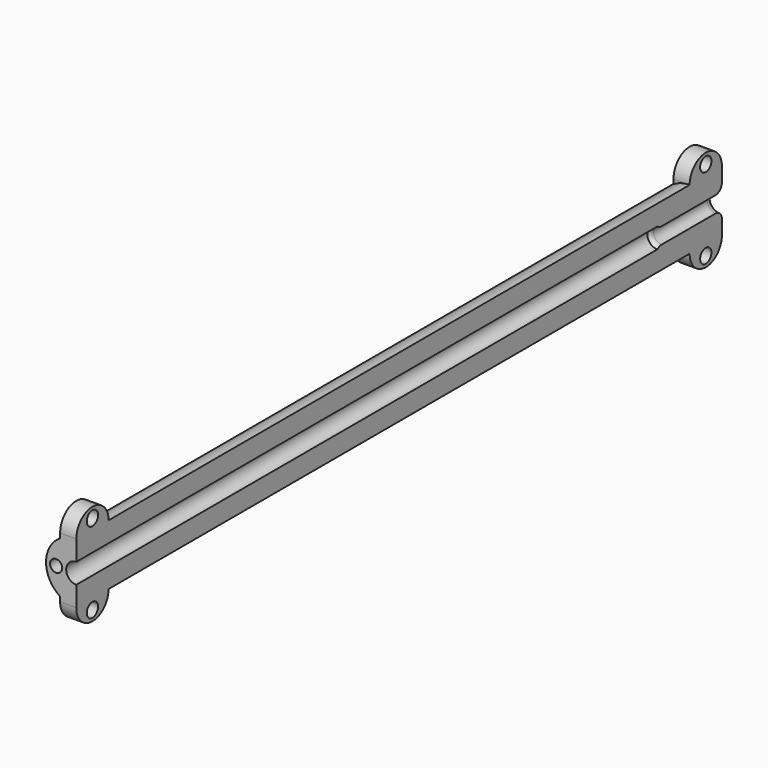
from build123d import *

# Parameters (mm, degrees)
F0_R         = 7.5
F0_R_2       = 2.5
F1_DEPTH     = 200
F2_R         = 1.5
F3_DEPTH     = 25
F4_W         = 255.6320726871
F4_H         = 34.7503256053
F5_DEPTH     = 25
F6_W         = 10
F6_H         = 5
F6_H_2       = 4.8793365061
F7_DEPTH     = 4
F8_R         = 1.75
F9_DEPTH     = 7.501
F11_DEPTH    = 20
F12_T2_ANGLE = 359.64
F12_T4_ANGLE = 359.64


# Not quite as in the source:
# - a fillet or chamfer that OpenCascade refuses, or shapes differently, is made with other operations: its cross-section is extruded or revolved along the edge and cut away or added


with BuildPart() as f1:
    # F0 (on Front) → F1 (new body)
    with BuildSketch(Plane.XZ):
        Circle(F0_R)
        Circle(F0_R_2, mode=Mode.SUBTRACT)
    extrude(amount=-F1_DEPTH)

    # F2 (on face) → F3 (cut)
    with BuildSketch(Plane.XZ):
        with Locations((5, 0)):
            Circle(F2_R)
        with Locations((-5, 0)):
            Circle(F2_R)
    extrude(amount=-F3_DEPTH, mode=Mode.SUBTRACT)

    # F4 (on Right) → F5 (cut)
    with BuildSketch(Plane.YZ):
        with Locations((127.8160363436, -0.9753750637)):
            Rectangle(F4_W, F4_H)
    extrude(amount=F5_DEPTH, mode=Mode.SUBTRACT)

    # F6 (on face) → F7 (join)
    with BuildSketch(Plane.YZ):
        with BuildLine():
            ThreePointArc((10, 7.5), (5, 12.5), (0, 7.5))
            Line((0, 7.5), (10, 7.5))
        make_face()
        with Locations((5, 5)):
            Rectangle(F6_W, F6_H)
        with BuildLine():
            Line((190, 7.5), (200, 7.5))
            ThreePointArc((200, 7.5), (195, 12.5), (190, 7.5))
        make_face()
        with Locations((195, 5)):
            Rectangle(F6_W, F6_H)
        with BuildLine():
            ThreePointArc((190, -7.5), (195, -12.5), (200, -7.5))
            Line((200, -7.5), (190, -7.5))
        make_face()
        with Locations((195, -5.0603317469)):
            Rectangle(F6_W, F6_H_2)
        with BuildLine():
            Line((10, -7.5), (0, -7.5))
            ThreePointArc((0, -7.5), (5, -12.5), (10, -7.5))
        make_face()
        with Locations((5, -5.0603317469)):
            Rectangle(F6_W, F6_H_2)
    extrude(amount=-F7_DEPTH)

    # F8 (on face) → F9 (cut, through all)
    with BuildSketch(Plane.YZ):
        with Locations((5, 10)):
            Circle(F8_R)
        with Locations((5, -10)):
            Circle(F8_R)
        with Locations((195, 10)):
            Circle(F8_R)
        with Locations((195, -10)):
            Circle(F8_R)
    extrude(amount=-F9_DEPTH, mode=Mode.SUBTRACT)

    # F10 (on face) → F11 (join)
    with BuildSketch(Plane(origin=(0, 200, 0), x_dir=(-1, 0, 0), z_dir=(0, 1, 0))):
        with BuildLine():
            Line((0, 2.5), (0, 2))
            ThreePointArc((0, 2), (2, 0), (0, -2))
            Line((0, -2), (0, -2.5))
            ThreePointArc((0, -2.5), (2.5, 0), (0, 2.5))
        make_face()
    extrude(amount=-F11_DEPTH)

    # F12: fillet of radius 2 on 2 edges, made by hand

    # F12_s1 → F12_t2 (revolve, cut)
    with BuildSketch(Plane(origin=(0, 0, 0), x_dir=(0, 1, 0), z_dir=(0.0031415875, 0, -0.9999950652))):
        with BuildLine():
            ThreePointArc((198, 2), (199.4142135624, 2.5857864376), (200, 4))
            Line((200, 4), (200, 2))
            Line((200, 2), (198, 2))
        make_face()
    revolve(axis=Axis((0, 200, 0), (0, -1, 0)), revolution_arc=F12_T2_ANGLE, mode=Mode.SUBTRACT)

    # F12_s3 → F12_t4 (revolve, cut)
    with BuildSketch(Plane(origin=(0, 0, 0), x_dir=(0, 1, 0), z_dir=(0.0031415875, 0, -0.9999950652))):
        with BuildLine():
            ThreePointArc((180, 2.5), (180.6157688743, 2.1291713066), (181.3228756555, 2))
            Line((181.3228756555, 2), (180, 2))
            Line((180, 2), (180, 2.5))
        make_face()
    revolve(axis=Axis((0, 180, 0), (0, -1, 0)), revolution_arc=F12_T4_ANGLE, mode=Mode.SUBTRACT)


solid = f1.part
